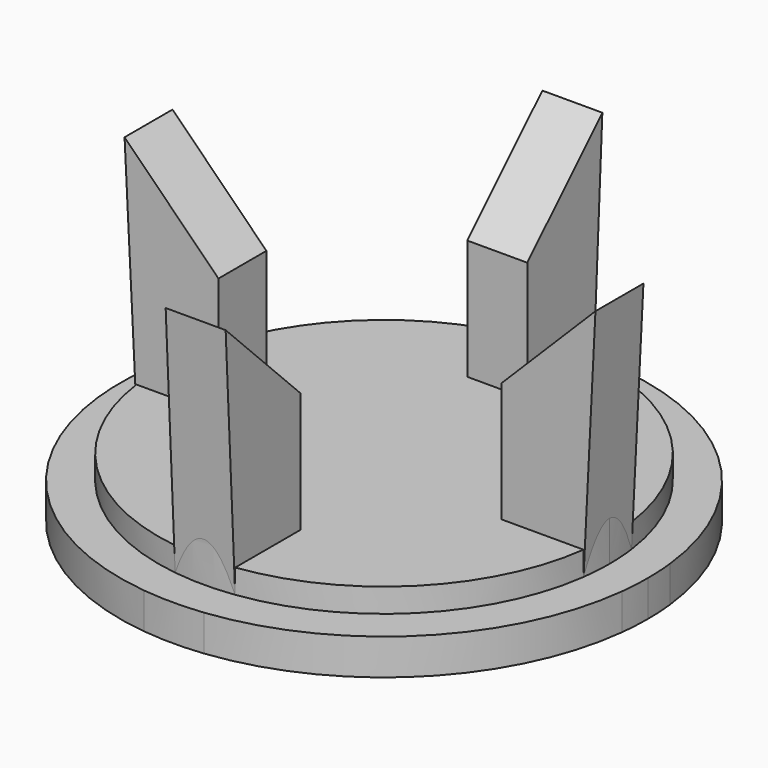
from build123d import *

# Parameters (mm, degrees)
F1_DEPTH     = 1.5
F2_DEPTH     = 10
F4_DEPTH     = 2.5
F6_DEPTH     = 2.5
F8_DEPTH     = 2.5
F10_DEPTH    = 2.5
F11_DEPTH    = 1
F12_T1_DEPTH = 23.0734639037
F12_T3_DEPTH = 23.0734639037


# Not quite as in the source:
# - a fillet or chamfer that OpenCascade refuses, or shapes differently, is made with other operations: its cross-section is extruded or revolved along the edge and cut away or added


with BuildPart() as f1:
    # F0 (on Top) → F1 (new body)
    with BuildSketch(Plane.XY):
        with BuildLine():
            Line((-1.25, 9.3165175897), (-1.25, 10.9287464972))
            ThreePointArc((-1.25, 10.9287464972), (-7.7781745931, 7.7781745931), (-10.9287464972, 1.25))
            Line((-10.9287464972, 1.25), (-9.3165175897, 1.25))
            ThreePointArc((-9.3165175897, 1.25), (-6.6468037432, 6.6468037432), (-1.25, 9.3165175897))
        make_face()
        with BuildLine():
            ThreePointArc((-10.9287464972, -1.25), (-7.7781745931, -7.7781745931), (-1.25, -10.9287464972))
            Line((-1.25, -10.9287464972), (-1.25, -9.3165175897))
            ThreePointArc((-1.25, -9.3165175897), (-6.6468037432, -6.6468037432), (-9.3165175897, -1.25))
            Line((-9.3165175897, -1.25), (-10.9287464972, -1.25))
        make_face()
        with BuildLine():
            Line((-9.3165175897, 1.25), (-10.9287464972, 1.25))
            ThreePointArc((-10.9287464972, 1.25), (-11, 0), (-10.9287464972, -1.25))
            Line((-10.9287464972, -1.25), (-9.3165175897, -1.25))
            ThreePointArc((-9.3165175897, -1.25), (-9.4, 0), (-9.3165175897, 1.25))
        make_face()
        with BuildLine():
            ThreePointArc((1.25, -10.9287464972), (7.7781745931, -7.7781745931), (10.9287464972, -1.25))
            Line((10.9287464972, -1.25), (9.3165175897, -1.25))
            ThreePointArc((9.3165175897, -1.25), (6.6468037432, -6.6468037432), (1.25, -9.3165175897))
            Line((1.25, -9.3165175897), (1.25, -10.9287464972))
        make_face()
        with BuildLine():
            ThreePointArc((-1.25, -10.9287464972), (0, -11), (1.25, -10.9287464972))
            Line((1.25, -10.9287464972), (1.25, -9.3165175897))
            ThreePointArc((1.25, -9.3165175897), (0, -9.4), (-1.25, -9.3165175897))
            Line((-1.25, -9.3165175897), (-1.25, -10.9287464972))
        make_face()
        with BuildLine():
            Line((9.3165175897, 1.25), (10.9287464972, 1.25))
            ThreePointArc((10.9287464972, 1.25), (7.7781745931, 7.7781745931), (1.25, 10.9287464972))
            Line((1.25, 10.9287464972), (1.25, 9.3165175897))
            ThreePointArc((1.25, 9.3165175897), (6.6468037432, 6.6468037432), (9.3165175897, 1.25))
        make_face()
        with BuildLine():
            ThreePointArc((10.9287464972, -1.25), (10.9821721774, -0.6260145888), (11, 0))
            ThreePointArc((11, 0), (10.9821721774, 0.6260145888), (10.9287464972, 1.25))
            Line((10.9287464972, 1.25), (9.3165175897, 1.25))
            ThreePointArc((9.3165175897, 1.25), (9.3791061766, 0.6263923117), (9.4, 0))
            ThreePointArc((9.4, 0), (9.3791061766, -0.6263923117), (9.3165175897, -1.25))
            Line((9.3165175897, -1.25), (10.9287464972, -1.25))
        make_face()
        with BuildLine():
            Line((1.25, 9.3165175897), (1.25, 10.9287464972))
            ThreePointArc((1.25, 10.9287464972), (0, 11), (-1.25, 10.9287464972))
            Line((-1.25, 10.9287464972), (-1.25, 9.3165175897))
            ThreePointArc((-1.25, 9.3165175897), (0, 9.4), (1.25, 9.3165175897))
        make_face()
        with BuildLine():
            Line((5.9, 1.25), (9.3165175897, 1.25))
            ThreePointArc((9.3165175897, 1.25), (6.6468037432, 6.6468037432), (1.25, 9.3165175897))
            Line((1.25, 9.3165175897), (1.25, 5.9))
            Line((1.25, 5.9), (-1.25, 5.9))
            Line((-1.25, 5.9), (-1.25, 9.3165175897))
            ThreePointArc((-1.25, 9.3165175897), (-6.6468037432, 6.6468037432), (-9.3165175897, 1.25))
            Line((-9.3165175897, 1.25), (-5.9, 1.25))
            Line((-5.9, 1.25), (-5.9, -1.25))
            Line((-5.9, -1.25), (-9.3165175897, -1.25))
            ThreePointArc((-9.3165175897, -1.25), (-6.6468037432, -6.6468037432), (-1.25, -9.3165175897))
            Line((-1.25, -9.3165175897), (-1.25, -5.9))
            Line((-1.25, -5.9), (1.25, -5.9))
            Line((1.25, -5.9), (1.25, -9.3165175897))
            ThreePointArc((1.25, -9.3165175897), (6.6468037432, -6.6468037432), (9.3165175897, -1.25))
            Line((9.3165175897, -1.25), (5.9, -1.25))
            Line((5.9, -1.25), (5.9, 1.25))
        make_face()
        with BuildLine():
            Line((1.25, 5.9), (1.25, 9.3165175897))
            ThreePointArc((1.25, 9.3165175897), (0, 9.4), (-1.25, 9.3165175897))
            Line((-1.25, 9.3165175897), (-1.25, 5.9))
            Line((-1.25, 5.9), (1.25, 5.9))
        make_face()
        with BuildLine():
            ThreePointArc((9.4, 0), (9.3791061766, 0.6263923117), (9.3165175897, 1.25))
            Line((9.3165175897, 1.25), (5.9, 1.25))
            Line((5.9, 1.25), (5.9, -1.25))
            Line((5.9, -1.25), (9.3165175897, -1.25))
            ThreePointArc((9.3165175897, -1.25), (9.3791061766, -0.6263923117), (9.4, 0))
        make_face()
        with BuildLine():
            Line((-5.9, 1.25), (-9.3165175897, 1.25))
            ThreePointArc((-9.3165175897, 1.25), (-9.4, 0), (-9.3165175897, -1.25))
            Line((-9.3165175897, -1.25), (-5.9, -1.25))
            Line((-5.9, -1.25), (-5.9, 1.25))
        make_face()
        with BuildLine():
            ThreePointArc((-1.25, -9.3165175897), (0, -9.4), (1.25, -9.3165175897))
            Line((1.25, -9.3165175897), (1.25, -5.9))
            Line((1.25, -5.9), (-1.25, -5.9))
            Line((-1.25, -5.9), (-1.25, -9.3165175897))
        make_face()
    extrude(amount=-F1_DEPTH)

    # F0 (on Top) → F2 (join)
    with BuildSketch(Plane.XY):
        with BuildLine():
            Line((1.25, 5.9), (1.25, 9.3165175897))
            ThreePointArc((1.25, 9.3165175897), (0, 9.4), (-1.25, 9.3165175897))
            Line((-1.25, 9.3165175897), (-1.25, 5.9))
            Line((-1.25, 5.9), (1.25, 5.9))
        make_face()
        with BuildLine():
            ThreePointArc((9.4, 0), (9.3791061766, 0.6263923117), (9.3165175897, 1.25))
            Line((9.3165175897, 1.25), (5.9, 1.25))
            Line((5.9, 1.25), (5.9, -1.25))
            Line((5.9, -1.25), (9.3165175897, -1.25))
            ThreePointArc((9.3165175897, -1.25), (9.3791061766, -0.6263923117), (9.4, 0))
        make_face()
        with BuildLine():
            Line((-5.9, 1.25), (-9.3165175897, 1.25))
            ThreePointArc((-9.3165175897, 1.25), (-9.4, 0), (-9.3165175897, -1.25))
            Line((-9.3165175897, -1.25), (-5.9, -1.25))
            Line((-5.9, -1.25), (-5.9, 1.25))
        make_face()
        with BuildLine():
            ThreePointArc((-1.25, -9.3165175897), (0, -9.4), (1.25, -9.3165175897))
            Line((1.25, -9.3165175897), (1.25, -5.9))
            Line((1.25, -5.9), (-1.25, -5.9))
            Line((-1.25, -5.9), (-1.25, -9.3165175897))
        make_face()
    extrude(amount=F2_DEPTH)

    # F3 (on face) → F4 (join)
    with BuildSketch(Plane(origin=(-1.25, 0, 0), x_dir=(0, -1, 0), z_dir=(-1, 0, 0))):
        Polygon((-9.3165175897, 0), (-9.3165175897, 10), (-9.8165175897, 10), align=None)
    extrude(amount=-F4_DEPTH)

    # F5 (on face) → F6 (join)
    with BuildSketch(Plane(origin=(-1.25, 0, 0), x_dir=(0, -1, 0), z_dir=(-1, 0, 0))):
        Polygon((9.8165175897, 10), (9.3165175897, 10), (9.3165175897, 0), align=None)
    extrude(amount=-F6_DEPTH)

    # F7 (on face) → F8 (join)
    with BuildSketch(Plane.XZ.offset(1.25)):
        Polygon((-9.3165175897, 0), (-9.3165175897, 10), (-9.8165175897, 10), align=None)
    extrude(amount=-F8_DEPTH)

    # F9 (on face) → F10 (join)
    with BuildSketch(Plane.XZ.offset(1.25)):
        Polygon((9.8165175897, 10), (9.3165175897, 10), (9.3165175897, 0), align=None)
    extrude(amount=-F10_DEPTH)

    # F0 (on Top) → F11 (join)
    with BuildSketch(Plane.XY):
        with BuildLine():
            Line((5.9, 1.25), (9.3165175897, 1.25))
            ThreePointArc((9.3165175897, 1.25), (6.6468037432, 6.6468037432), (1.25, 9.3165175897))
            Line((1.25, 9.3165175897), (1.25, 5.9))
            Line((1.25, 5.9), (-1.25, 5.9))
            Line((-1.25, 5.9), (-1.25, 9.3165175897))
            ThreePointArc((-1.25, 9.3165175897), (-6.6468037432, 6.6468037432), (-9.3165175897, 1.25))
            Line((-9.3165175897, 1.25), (-5.9, 1.25))
            Line((-5.9, 1.25), (-5.9, -1.25))
            Line((-5.9, -1.25), (-9.3165175897, -1.25))
            ThreePointArc((-9.3165175897, -1.25), (-6.6468037432, -6.6468037432), (-1.25, -9.3165175897))
            Line((-1.25, -9.3165175897), (-1.25, -5.9))
            Line((-1.25, -5.9), (1.25, -5.9))
            Line((1.25, -5.9), (1.25, -9.3165175897))
            ThreePointArc((1.25, -9.3165175897), (6.6468037432, -6.6468037432), (9.3165175897, -1.25))
            Line((9.3165175897, -1.25), (5.9, -1.25))
            Line((5.9, -1.25), (5.9, 1.25))
        make_face()
    extrude(amount=F11_DEPTH)

    # F12: chamfer of 4 on 4 edges, made by hand

    # F12_s2 → F12_t1 (cut)
    with BuildSketch(Plane.YZ.offset(-11.5367319519)):
        Polygon((5.9, 6), (9.9, 10), (5.9, 10), align=None)
        Polygon((-9.9, 10), (-5.9, 6), (-5.9, 10), align=None)
    extrude(amount=F12_T1_DEPTH, mode=Mode.SUBTRACT)

    # F12_s4 → F12_t3 (cut)
    with BuildSketch(Plane.XZ.offset(-11.5367319519)):
        Polygon((9.9, 10), (5.9, 6), (5.9, 10), align=None)
        Polygon((-5.9, 6), (-9.9, 10), (-5.9, 10), align=None)
    extrude(amount=F12_T3_DEPTH, mode=Mode.SUBTRACT)


solid = f1.part
